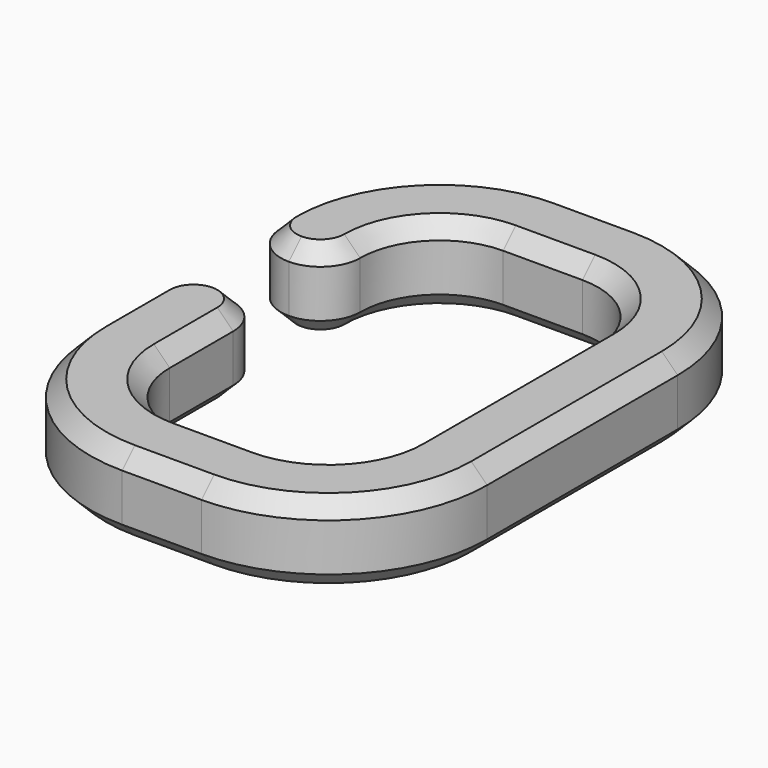
from build123d import *

# Parameters (mm, degrees)
F0_W     = 10
F0_H     = 15
F0_H_2   = 50
F0_H_3   = 25
F1_DEPTH = 10
F2_R     = 10
F3_R     = 20
F4_R     = 4.99999
F5_SIZE  = 2


# Not quite as in the source:
# - a fillet or chamfer is up to 0.001 mm smaller than in the source, because OpenCascade refuses the exact size


with BuildPart() as f1:
    # F0 (on Top) → F1 (new body)
    with BuildSketch(Plane.XY):
        with Locations((-40, 17.5)):
            Rectangle(F0_W, F0_H)
        Polygon((-35, 25), (-5, 25), (5, 25), (5, 35), (-45, 35), (-45, 25), align=None)
        Rectangle(F0_W, F0_H_2)
        Polygon((5, -25), (-5, -25), (-35, -25), (-45, -25), (-45, -35), (5, -35), align=None)
        with Locations((-40, -12.5)):
            Rectangle(F0_W, F0_H_3)
    extrude(amount=F1_DEPTH)

    # F2
    f2_edges = [f1.edges().sort_by_distance(p)[0] for p in [
        (-35, 25, 5),
        (-5, 25, 5),
        (-5, -25, 5),
        (-35, -25, 5),
    ]]
    fillet(f2_edges, radius=F2_R)

    # F3
    f3_edges = [f1.edges().sort_by_distance(p)[0] for p in [
        (5, 35, 5),
        (-45, 35, 5),
        (5, -35, 5),
        (-45, -35, 5),
    ]]
    fillet(f3_edges, radius=F3_R)

    # F4 (radius 5 in the source; OpenCascade refuses exactly that, so slightly less here)
    f4_edges = [f1.edges().sort_by_distance(p)[0] for p in [
        (-35, 10, 5),
        (-45, 10, 5),
        (-45, 0, 5),
        (-35, 0, 5),
    ]]
    fillet(f4_edges, radius=F4_R)

    # F5
    f5_edges = [f1.edges().sort_by_distance(p)[0] for p in [
        (-45, -9.999995, 0),
        (-39.142136, -29.142136, 10),
    ]]
    chamfer(f5_edges, length=F5_SIZE)


solid = f1.part
